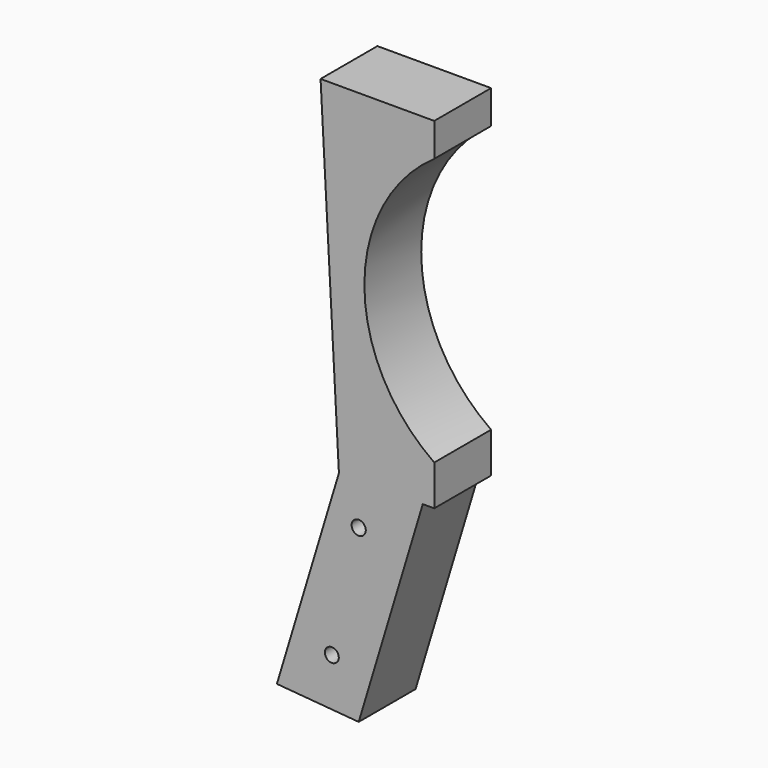
from build123d import *

# Parameters (mm, degrees)
F0_R     = 1.5571839485
F0_R_2   = 1.582453361
F1_DEPTH = 7.9375


# Not quite as in the source:
# - a feature names something its author has since deleted; it is built from what else it names


with BuildPart() as f1:
    # F0 (on Front) → F1 (new body, symmetric)
    with BuildSketch(Plane.XZ):
        with BuildLine():
            Line((-4.4244504534, -9.0134367347), (14.3148868547, -9.0134367347))
            Line((14.3148868547, -9.0134367347), (16.876486437, -9.0134367347))
            Line((16.876486437, -9.0134367347), (16.876486437, 0))
            ThreePointArc((16.876486437, 0), (1.2674691421, 29.8639013079), (16.876486437, 59.7278026158))
            Line((16.876486437, 59.7278026158), (16.876486437, 67.1865632653))
            Line((16.876486437, 67.1865632653), (-8.523513563, 67.1865632653))
            Line((-8.523513563, 67.1865632653), (-4.4244504534, -9.0134367347))
        make_face()
        Polygon((0, -56.506741792), (14.3148868547, -9.0134367347), (-4.4244504534, -9.0134367347), (-18.2776516019, -54.9749811636), align=None)
        with Locations((-6.0080750845, -45.2978610992)):
            Circle(F0_R, mode=Mode.SUBTRACT)
        with Locations((0, -18.3103610992)):
            Circle(F0_R_2, mode=Mode.SUBTRACT)
    extrude(amount=F1_DEPTH, both=True)


solid = f1.part
